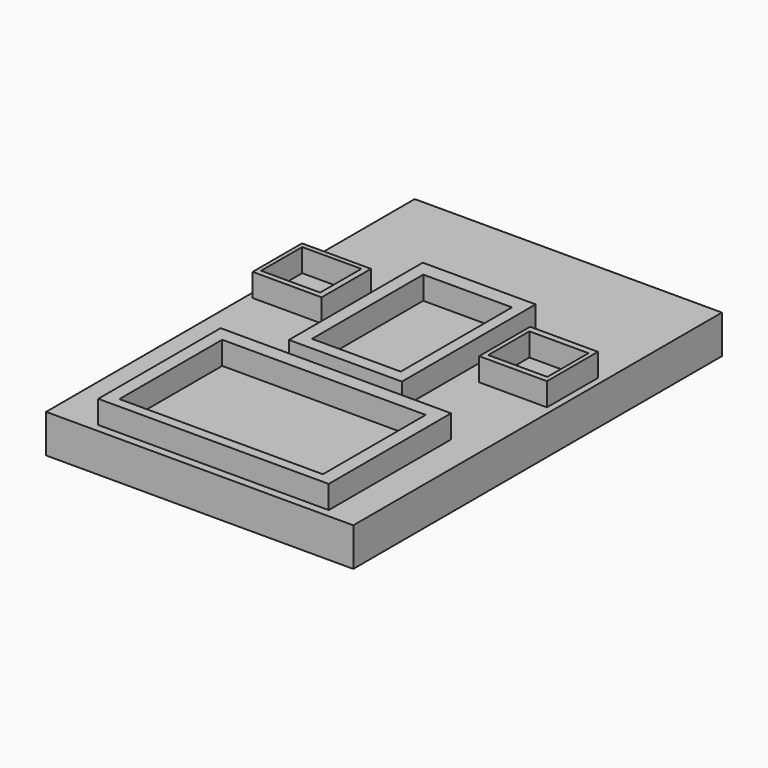
from build123d import *

# Parameters (mm, degrees)
F0_W     = 101.6
F0_H     = 152.4
F0_W_2   = 25.9637702256
F0_H_2   = 38.2640473545
F1_DEPTH = 12.7
F2_W     = 37.3481158167
F2_H     = 55.3146842867
F2_W_2   = 29.3511133641
F2_H_2   = 46.0022222251
F2_W_3   = 76.2175656855
F2_H_3   = 50.5883861333
F2_W_4   = 67.3006474972
F2_H_4   = 42.5056517124
F2_W_5   = 22.4156714976
F2_H_5   = 21.067361813
F2_W_6   = 19.5578802377
F2_H_6   = 17.0068526641
F2_W_7   = 22.81752415
F2_H_7   = 20.4082219861
F3_DEPTH = 7.62


with BuildPart() as f1:
    # F0 (on Top) → F1 (new body)
    with BuildSketch(Plane.XY):
        with Locations((-0.5644435562, 0)):
            Rectangle(F0_W, F0_H)
        with Locations((0.3079539165, 19.1320236772)):
            Rectangle(F0_W_2, F0_H_2, mode=Mode.SUBTRACT)
        with Locations((0.3079539165, 19.1320236772)):
            Rectangle(F0_W_2, F0_H_2)
    extrude(amount=F1_DEPTH)

    # F2 (on face) → F3 (join)
    with BuildSketch(Plane.XY.offset(12.7)):
        with Locations((0.2927491441, 10.6312921271)):
            Rectangle(F2_W, F2_H)
        with Locations((0.5644438788, 10.1600000635)):
            Rectangle(F2_W_2, F2_H_2, mode=Mode.SUBTRACT)
        with Locations((1.8496308476, -48.2227718458)):
            Rectangle(F2_W_3, F2_H_3)
        with Locations((1.7533935606, -48.9725470543)):
            Rectangle(F2_W_4, F2_H_4, mode=Mode.SUBTRACT)
        with Locations((36.8676688522, 17.0947427396)):
            Rectangle(F2_W_5, F2_H_5)
        with Locations((36.8869742379, 16.9948018156)):
            Rectangle(F2_W_6, F2_H_6, mode=Mode.SUBTRACT)
        with Locations((-38.0652910098, 17.0451246668)):
            Rectangle(F2_W_7, F2_H_7)
        with Locations((-38.3849483915, 17.1790141612)):
            Rectangle(F2_W_6, F2_H_6, mode=Mode.SUBTRACT)
    extrude(amount=F3_DEPTH)


solid = f1.part
